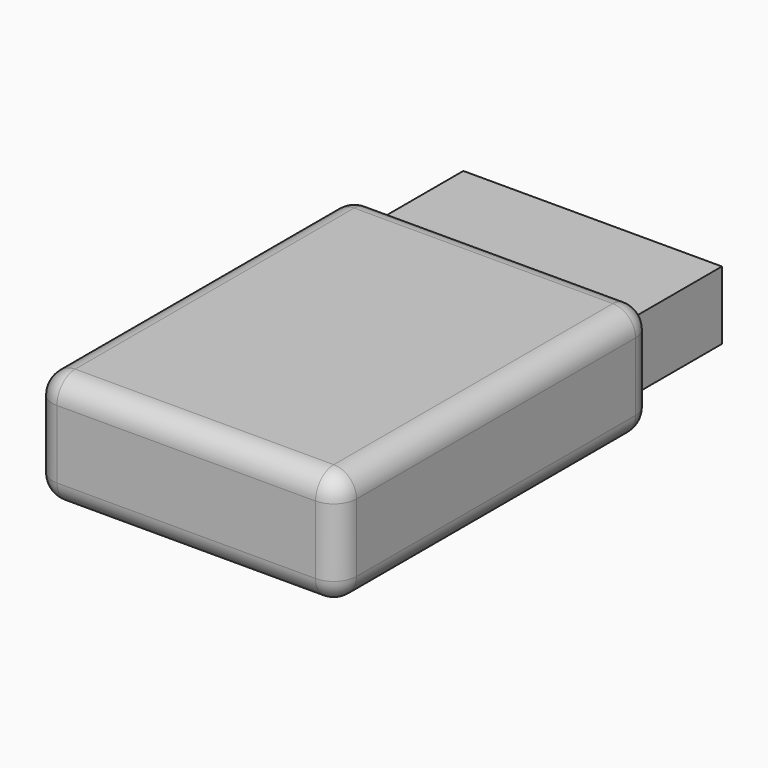
from build123d import *

# Parameters (mm, degrees)
F0_W     = 67.9279565811
F0_H     = 88.0647003651
F1_DEPTH = 25.4
F2_R     = 5.08
F3_DEPTH = 25.4
F4_W     = 52.0835686475
F4_H     = 10.6304162182
F5_DEPTH = 25.4


# Not quite as in the source:
# - a feature of the source that left no trace in its solid (it failed there, or was rolled back) is left out


with BuildPart() as f1:
    # F0 (on Top) → F1 (new body)
    with BuildSketch(Plane.XY):
        Rectangle(F0_W, F0_H)
    extrude(amount=F1_DEPTH)

    # F2
    f2_edges = [f1.edges().sort_by_distance(p)[0] for p in [
        (33.963978, -44.03235, 12.7),
        (33.963978, 44.03235, 12.7),
        (33.963978, 0, 0),
        (33.963978, 0, 25.4),
        (-33.963978, -44.03235, 12.7),
        (0, -44.03235, 0),
        (0, -44.03235, 25.4),
        (-33.963978, 44.03235, 12.7),
        (-33.963978, 0, 0),
        (-33.963978, 0, 25.4),
        (0, 44.03235, 0),
        (0, 44.03235, 25.4),
    ]]
    fillet(f2_edges, radius=F2_R)

    # F3 (add): a face of the model
    f3_faces = [f1.faces().sort_by_distance(p)[0] for p in [
        (0, 44.0323501825, 12.7),
    ]]
    extrude(f3_faces, amount=F3_DEPTH)

    # F4 (on face) → F5 (cut)
    with BuildSketch(Plane(origin=(0, 69.4323501825, 0), x_dir=(-1, 0, 0), z_dir=(0, 1, 0))):
        with Locations((0.3008237109, 12.2958261054)):
            Rectangle(F4_W, F4_H)
    extrude(amount=-F5_DEPTH, mode=Mode.SUBTRACT)


solid = f1.part
